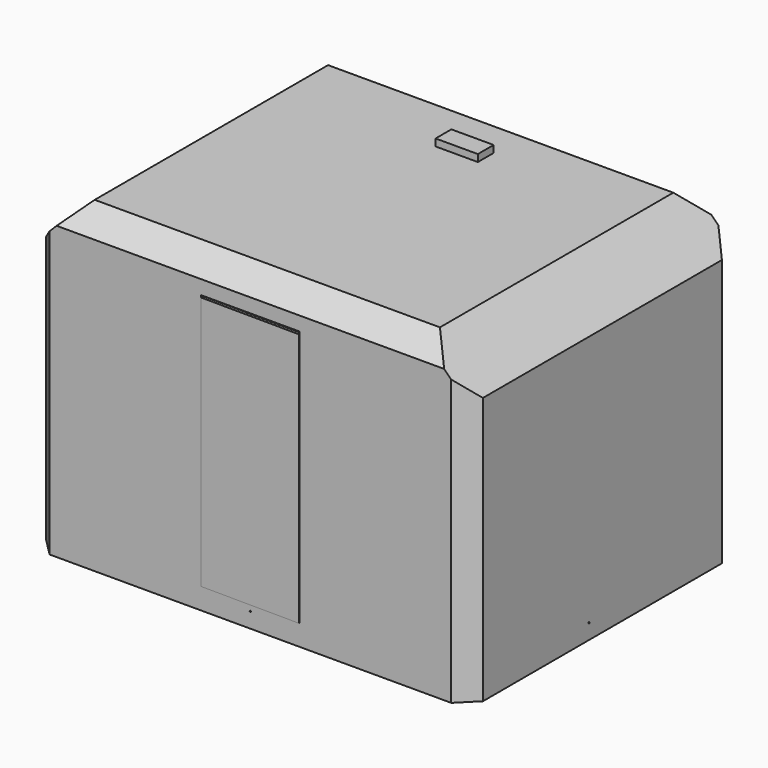
from build123d import *

# Parameters (mm, degrees)
F0_W           = 3100
F0_H           = 2220
F1_DEPTH       = 2370
F2_SIZE        = 325
F3_SIZE        = 325
F4_SIZE        = 125
F5_SIZE        = 125
F6_SIZE        = 125
F7_SIZE        = 125
F8_W           = 1519
F8_H           = 1519
F9_DEPTH       = 108
F10_W          = 400
F10_H          = 200
F10_R          = 7.5
F11_DEPTH      = 1
F12_R          = 5
F13_DEPTH      = 1
F14_DEPTH      = 790.501
F14_DEPTH_BACK = 2309.501
F15_R          = 5
F16_DEPTH      = 545.001
F16_DEPTH_BACK = 1825.001
F17_SIZE       = 150
F18_SIZE       = 150
F19_W          = 1719
F19_H          = 1719
F19_W_2        = 1519
F19_H_2        = 1519
F20_DEPTH      = 15
F21_W          = 700
F21_H          = 1820
F22_DEPTH      = 20
F23_W          = 300
F23_H          = 140
F24_DEPTH      = 50
F26_DEPTH      = 1805


# Not quite as in the source:
# - a feature of the source that left no trace in its solid (it failed there, or was rolled back) is left out


with BuildPart() as f1:
    # F0 (on Front) → F1 (new body)
    with BuildSketch(Plane.XZ):
        Rectangle(F0_W, F0_H)
    extrude(amount=F1_DEPTH)

    # F2
    f2_edges = [f1.edges().sort_by_distance(p)[0] for p in [
        (-1550, -1185, 1110),
    ]]
    chamfer(f2_edges, length=F2_SIZE)

    # F3
    f3_edges = [f1.edges().sort_by_distance(p)[0] for p in [
        (1550, -1185, 1110),
    ]]
    chamfer(f3_edges, length=F3_SIZE)

    # F4
    f4_edges = [f1.edges().sort_by_distance(p)[0] for p in [
        (1550, -2370, -162.5),
    ]]
    chamfer(f4_edges, length=F4_SIZE)

    # F5
    f5_edges = [f1.edges().sort_by_distance(p)[0] for p in [
        (-1550, -2370, -162.5),
    ]]
    chamfer(f5_edges, length=F5_SIZE)

    # F6
    f6_edges = [f1.edges().sort_by_distance(p)[0] for p in [
        (-1550, 0, -162.5),
    ]]
    chamfer(f6_edges, length=F6_SIZE)

    # F7
    f7_edges = [f1.edges().sort_by_distance(p)[0] for p in [
        (1550, 0, -162.5),
    ]]
    chamfer(f7_edges, length=F7_SIZE)

    # F8 (on face) → F9 (cut)
    with BuildSketch(Plane(origin=(0, 0, -1110), x_dir=(1, 0, 0), z_dir=(0, 0, -1))):
        with Locations((0, 1304.5)):
            Rectangle(F8_W, F8_H)
    extrude(amount=-F9_DEPTH, mode=Mode.SUBTRACT)

    # F10 (on face) → F11 (cut)
    with BuildSketch(Plane(origin=(0, 0, -1002), x_dir=(1, 0, 0), z_dir=(0, 0, -1))):
        with Locations((0, 1854)):
            Rectangle(F10_W, F10_H)
        with Locations((0, 1934)):
            Circle(F10_R, mode=Mode.SUBTRACT)
        Polygon((601.4287087912, 1258.7050807569), (428.2236280343, 1358.7050807569), (228.2236280343, 1012.2949192431), (401.4287087912, 912.2949192431), align=None)
        with Locations((484.1082007155, 1095.5)):
            Circle(F10_R, mode=Mode.SUBTRACT)
        Polygon((-228.2236280343, 1012.2949192431), (-428.2236280343, 1358.7050807569), (-601.4287087912, 1258.7050807569), (-401.4287087912, 912.2949192431), align=None)
        with Locations((-484.1082007155, 1095.5)):
            Circle(F10_R, mode=Mode.SUBTRACT)
        with Locations((0, 1375)):
            Circle(F10_R)
    extrude(amount=-F11_DEPTH, mode=Mode.SUBTRACT)

    # F12 (on face) → F13 (cut)
    with BuildSketch(Plane.YZ.offset(-759.5)):
        with Locations((-1304.5, -1002)):
            Circle(F12_R)
    extrude(amount=F13_DEPTH, mode=Mode.SUBTRACT)

    # F12 (on face) → F14 (cut, two sides)
    with BuildSketch(Plane.YZ.offset(-759.5)) as f14_sk:
        with Locations((-1304.5, -1002)):
            Circle(F12_R)
    extrude(amount=-F14_DEPTH, mode=Mode.SUBTRACT)
    extrude(f14_sk.sketch, amount=F14_DEPTH_BACK, mode=Mode.SUBTRACT)

    # F15 (on face) → F16 (cut, two sides)
    with BuildSketch(Plane.XZ.offset(545)) as f16_sk:
        with Locations((0, -1002)):
            Circle(F15_R)
    extrude(amount=-F16_DEPTH, mode=Mode.SUBTRACT)
    extrude(f16_sk.sketch, amount=F16_DEPTH_BACK, mode=Mode.SUBTRACT)

    # F17
    f17_edges = [f1.edges().sort_by_distance(p)[0] for p in [
        (0, 0, 1110),
    ]]
    chamfer(f17_edges, length=F17_SIZE)

    # F18
    f18_edges = [f1.edges().sort_by_distance(p)[0] for p in [
        (0, -2370, 1110),
    ]]
    chamfer(f18_edges, length=F18_SIZE)

    # F19 (on face) → F20 (join)
    with BuildSketch(Plane(origin=(0, 0, -1110), x_dir=(1, 0, 0), z_dir=(0, 0, -1))):
        with Locations((0, 1304.5)):
            Rectangle(F19_W, F19_H)
        with Locations((0, 1304.5)):
            Rectangle(F19_W_2, F19_H_2, mode=Mode.SUBTRACT)
    extrude(amount=F20_DEPTH)

    # F21 (on face) → F22 (cut)
    with BuildSketch(Plane.XZ.offset(2370)):
        with Locations((0, -50)):
            Rectangle(F21_W, F21_H)
    extrude(amount=-F22_DEPTH, mode=Mode.SUBTRACT)

    # F23 (on face) → F24 (join)
    with BuildSketch(Plane.XY.offset(1110)):
        with Locations((0, -470)):
            Rectangle(F23_W, F23_H)
    extrude(amount=F24_DEPTH)

    # F25 (on face) → F26 (join)
    with BuildSketch(Plane.XY.offset(-960)):
        Polygon((-350, -2350), (-350.17453071, -2369.9992384613), (349.798815435, -2376.1078133101), (349.9733461449, -2356.1085748489), align=None)
    extrude(amount=F26_DEPTH)


solid = f1.part
